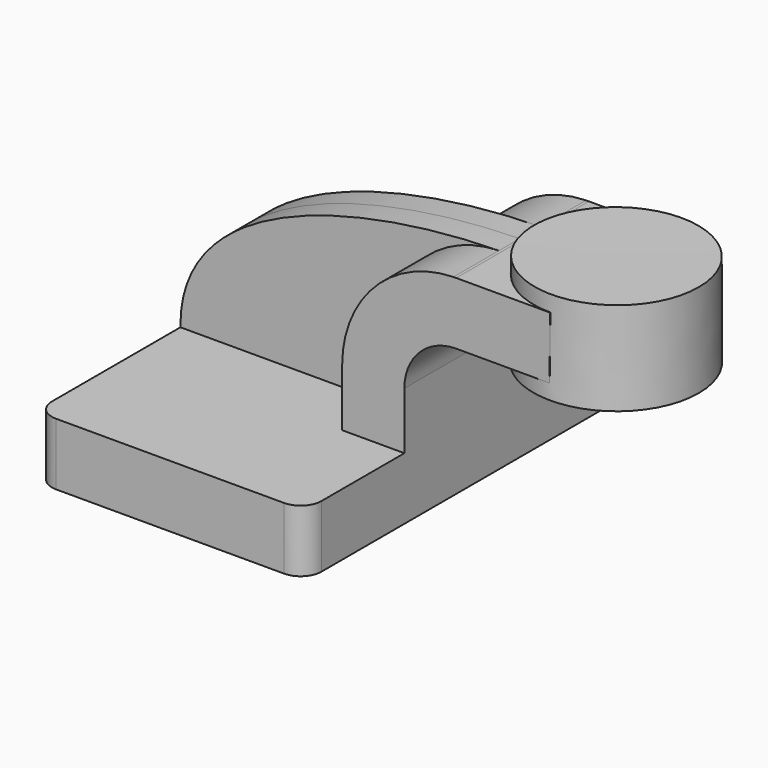
from build123d import *

# Parameters (mm, degrees)
F1_DEPTH = 63.5
F2_DEPTH = 25.4
F3_DEPTH = 7.9375
F5_R     = 6.35


with BuildPart() as f1:
    # F0 (on Front) → F1 (new body, symmetric)
    with BuildSketch(Plane.XZ):
        Polygon((22.225, 9.525), (-41.275, 9.525), (-41.275, -9.525), (41.275, -9.525), (41.275, 9.525), align=None)
    extrude(amount=F1_DEPTH, both=True)

    # F0 (on Front) → F2 (join, symmetric)
    with BuildSketch(Plane.XZ):
        with BuildLine():
            Line((22.225, 27.0002), (22.225, 9.525))
            Line((22.225, 9.525), (41.275, 9.525))
            Line((41.275, 9.525), (41.275, 27.0002))
            ThreePointArc((41.275, 27.0002), (45.9246798487, 38.2255201513), (57.15, 42.8752))
            Line((57.15, 42.8752), (60.325, 42.8752))
            Line((60.325, 42.8752), (60.325, 61.9252))
            Line((60.325, 61.9252), (57.15, 61.9252))
            add(Edge.make_bspline(
                [(56.2807505005, 61.9143809342), (56.5712025295, 61.918597831), (56.8609603005, 61.9222027986), (57.15, 61.9252)],
                knots=[110.7360058155, 110.7360058155, 110.7360058155, 110.7360058155, 111.5045361635, 111.5045361635, 111.5045361635, 111.5045361635], degree=3))
            ThreePointArc((56.2807505005, 61.9143809342), (32.1488583884, 51.3866417887), (22.225, 27.0002))
        make_face()
        Polygon((85.8728378947, 61.9252), (60.325, 61.9252), (60.325, 42.8752), (85.7546306228, 42.8752), align=None)
    extrude(amount=F2_DEPTH, both=True)

    # F0 (on Front) → F3 (join, symmetric)
    with BuildSketch(Plane.XZ):
        with BuildLine():
            add(Edge.make_bspline(
                [(-41.275, 9.525), (-41.8342912286, 47.9946959392), (14.430096654, 61.3067766904), (56.2807505005, 61.9143809342)],
                knots=[0, 0, 0, 0, 110.7360058155, 110.7360058155, 110.7360058155, 110.7360058155], degree=3))
            Line((-41.275, 9.525), (22.225, 9.525))
            Line((22.225, 9.525), (22.225, 27.0002))
            ThreePointArc((22.225, 27.0002), (32.1488583884, 51.3866417887), (56.2807505005, 61.9143809342))
        make_face()
    extrude(amount=F3_DEPTH, both=True)

    # F0 (on Front) → F4 (revolve)
    with BuildSketch(Plane.XZ):
        Polygon((85.9023109078, 66.675), (85.8728378947, 61.9252), (85.7546306228, 42.8752), (85.725, 38.1), (111.125, 38.1), (111.125, 66.675), align=None)
    revolve(axis=Axis((85.8136554539, 0, 52.3875), (0.0062049867, 0, 0.9999807489)))

    # F5
    f5_edges = [f1.edges().sort_by_distance(p)[0] for p in [
        (41.275, -63.5, 0),
        (41.275, 63.5, 0),
        (-41.275, 63.5, 0),
        (-41.275, -63.5, 0),
    ]]
    fillet(f5_edges, radius=F5_R)


solid = f1.part
